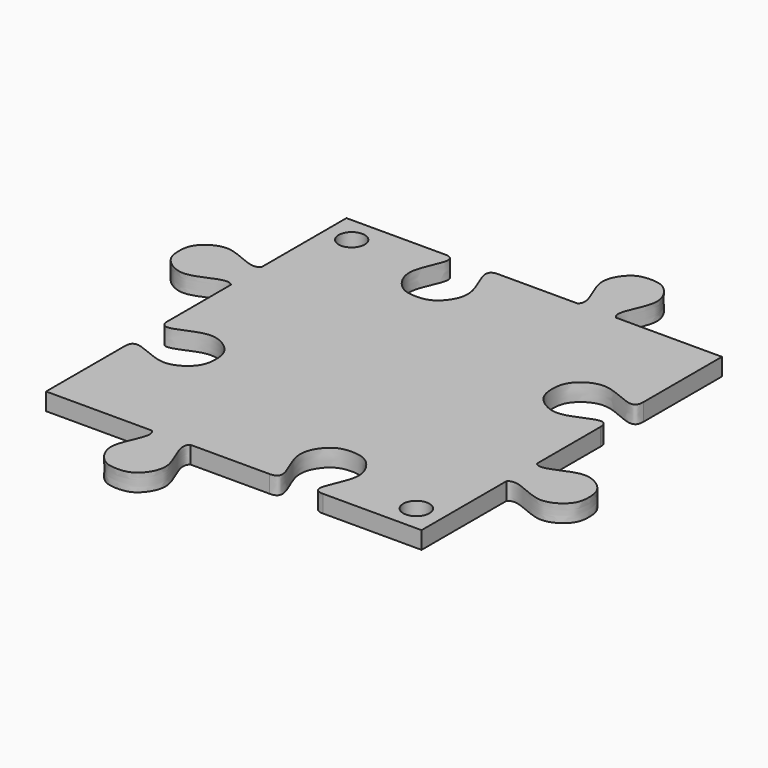
from build123d import *

# Parameters (mm, degrees)
F0_W            = 68.58
F0_H            = 68.58
F0_R            = 2.38125
F1_DEPTH        = 3.175
F3_DEPTH        = 3.175
F3_COPIES_COUNT = 4
F5_DEPTH        = 3.1760001
F5_COPIES_COUNT = 4


# Not quite as in the source:
# - ends of sketch curves that miss each other by under 0.0002 mm in the source are joined
# - the dataset's text gives a spline's control points without its knots; the knots are read off the source's solid
# - a pattern or mirror of a feature is missing from the dataset's text; its kind, count and spacing are read off the source's solid


with BuildPart() as f1:
    # F0 (on Top) → F1 (new body)
    with BuildSketch(Plane.XY):
        Rectangle(F0_W, F0_H)
        with Locations((29.5275, -29.5275)):
            Circle(F0_R, mode=Mode.SUBTRACT)
        with Locations((-29.5275, 29.5275)):
            Circle(F0_R, mode=Mode.SUBTRACT)
    extrude(amount=F1_DEPTH)

    # F2 (on Top) → F3 (join, through all)
    with BuildSketch(Plane.XY):
        with BuildLine():
            Line((-34.29, 7.915765397), (-34.29, 14.944234603))
            add(Edge.make_bspline(
                [(-34.29, 14.944234603), (-34.3313558628, 14.8935785161), (-34.4426172531, 14.7768003738), (-34.7268569626, 14.5791767248), (-35.1632825828, 14.4610729687), (-35.6905615765, 14.4797732889), (-36.2242014243, 14.5907562015), (-36.7635149779, 14.7564225299), (-37.4990555845, 15.0301487796), (-38.4432106763, 15.4359466178), (-39.5958051595, 15.9162128956), (-40.5443835243, 16.2215854131), (-41.2767903216, 16.3594127772), (-41.8045682937, 16.3979759573), (-42.322321412, 16.36635202), (-42.9986151142, 16.241576546), (-43.8064226218, 15.9455557367), (-44.6779218088, 15.4228004743), (-45.2894576242, 14.8978069093), (-45.6877742031, 14.4613491188), (-46.0224390664, 14.0146085438), (-46.3338924299, 13.414733443), (-46.5583124021, 12.5523976438), (-46.609, 11.8339160129), (-46.609, 11.43)],
                knots=[0.0676191782, 0.0676191782, 0.0676191782, 0.0676191782, 0.078125, 0.09375, 0.125, 0.15625, 0.1875, 0.21875, 0.25, 0.3125, 0.375, 0.4375, 0.46875, 0.5, 0.53125, 0.5625, 0.625, 0.6875, 0.75, 0.78125, 0.8125, 0.875, 0.9375, 1, 1, 1, 1], degree=3))
            add(Edge.make_bspline(
                [(-34.29, 7.915765397), (-34.3313558628, 7.9664214839), (-34.4426172531, 8.0831996262), (-34.7268569626, 8.2808232752), (-35.1632825828, 8.3989270313), (-35.6905615765, 8.3802267111), (-36.2242014243, 8.2692437985), (-36.7635149779, 8.1035774701), (-37.4990555845, 7.8298512204), (-38.4432106763, 7.4240533822), (-39.5958051595, 6.9437871044), (-40.5443835243, 6.6384145869), (-41.2767903216, 6.5005872228), (-41.8045682937, 6.4620240427), (-42.322321412, 6.49364798), (-42.9986151142, 6.618423454), (-43.8064226218, 6.9144442633), (-44.6779218088, 7.4371995257), (-45.2894576242, 7.9621930907), (-45.6877742031, 8.3986508812), (-46.0224390664, 8.8453914562), (-46.3338924299, 9.445266557), (-46.5583124021, 10.3076023562), (-46.609, 11.0260839871), (-46.609, 11.43)],
                knots=[0.0676191782, 0.0676191782, 0.0676191782, 0.0676191782, 0.078125, 0.09375, 0.125, 0.15625, 0.1875, 0.21875, 0.25, 0.3125, 0.375, 0.4375, 0.46875, 0.5, 0.53125, 0.5625, 0.625, 0.6875, 0.75, 0.78125, 0.8125, 0.875, 0.9375, 1, 1, 1, 1], degree=3))
        make_face()
    f3 = extrude(amount=F3_DEPTH)

    # F3_copies: F3 ×4 about axis
    f3_copies_axis = Axis((0, 0, 0), (0, 0, 1))
    for i in range(1, F3_COPIES_COUNT):
        add(f3.rotate(f3_copies_axis, i * 360 / F3_COPIES_COUNT))

    # F2 (on Top) → F5 (cut, through all)
    with BuildSketch(Plane.XY):
        with BuildLine():
            Line((39.124917239, 16.3318022102), (34.29, 16.3318022102))
            add(Edge.make_bspline(
                [(34.29, 16.3318022102), (34.29, 14.7647648175), (32.0429656083, 14.6161879321), (27.0096484518, 17.8052486363), (22.4209826376, 15.1763363508), (21.59, 13.066948405), (21.59, 11.43)],
                knots=[0, 0, 0, 0, 0.1915483917, 0.4921212841, 0.7562809095, 1, 1, 1, 1], degree=3))
            add(Edge.make_bspline(
                [(34.29, 6.5281977898), (34.29, 8.0952351825), (32.0429656083, 8.2438120679), (27.0096484518, 5.0547513637), (22.4209826376, 7.6836636492), (21.59, 9.793051595), (21.59, 11.43)],
                knots=[0, 0, 0, 0, 0.1915483917, 0.4921212841, 0.7562809095, 1, 1, 1, 1], degree=3))
            Line((34.29, 6.5281977898), (39.124917239, 6.5281977898))
            Line((39.124917239, 6.5281977898), (39.124917239, 16.3318022102))
        make_face()
    f5 = extrude(amount=F5_DEPTH, mode=Mode.SUBTRACT)

    # F5_copies: F5 ×4 about axis
    f5_copies_axis = Axis((0, 0, 0), (0, 0, 1))
    for i in range(1, F5_COPIES_COUNT):
        add(f5.rotate(f5_copies_axis, i * 360 / F5_COPIES_COUNT), mode=Mode.SUBTRACT)


solid = f1.part
